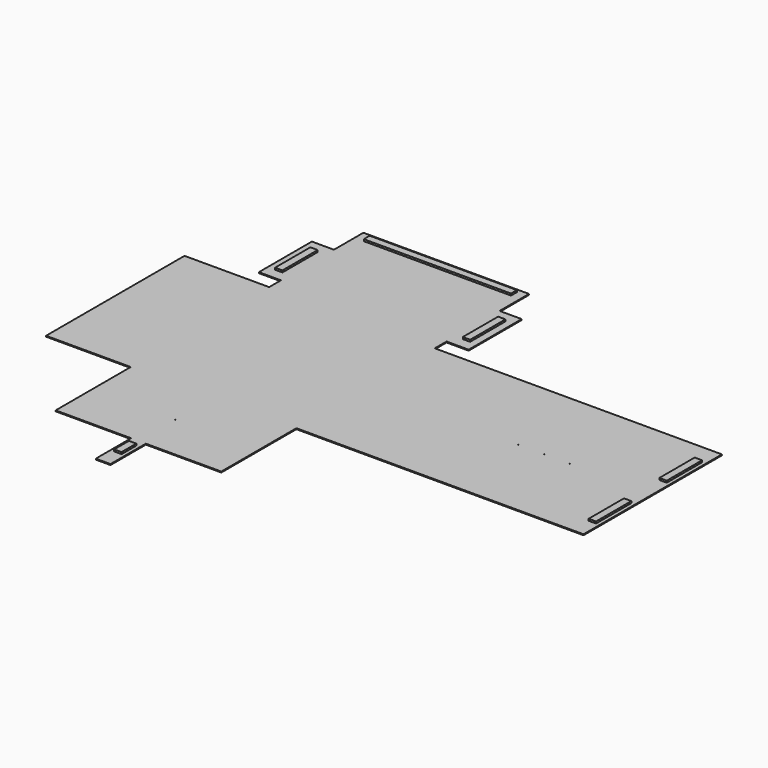
from build123d import *

# Parameters (mm, degrees)
F0_R      = 0.635
F1_DEPTH  = 3.175
F2_W      = 508
F2_H      = 25.4
F3_DEPTH  = 6.35
F4_W      = 25.4
F4_H      = 63.5
F4_H_2    = 152.4
F5_DEPTH  = 6.35
F6_W      = 508
F6_H      = 25.4
F7_DEPTH  = 6.35
F8_W      = 152.4
F8_H      = 25.4
F9_DEPTH  = 6.35
F10_W     = 25.4
F10_H     = 152.4
F11_DEPTH = 6.35
F12_W     = 25.4
F12_H     = 152.4
F13_DEPTH = 6.35
F14_W     = 76.2
F14_H     = 25.4
F15_DEPTH = 6.35


# Not quite as in the source:
# - a feature of the source that left no trace in its solid (it failed there, or was rolled back) is left out


with BuildPart() as f1:
    # F0 (on Top) → F1 (new body)
    with BuildSketch(Plane.XY):
        Polygon((285.75, -298.45), (323.85, -298.45), (577.85, -298.45), (615.95, -298.45), (1187.45, -298.45), (1276.35, -298.45), (1276.35, 298.45), (1187.45, 298.45), (285.75, 298.45), (285.75, 349.25), (361.95, 349.25), (361.95, 577.85), (285.75, 577.85), (285.75, 704.85), (-285.75, 704.85), (-285.75, 577.85), (-361.95, 577.85), (-361.95, 349.25), (-285.75, 349.25), (-285.75, 336.55), (-285.75, 298.45), (-323.85, 298.45), (-361.95, 298.45), (-577.85, 298.45), (-577.85, -298.45), (-323.85, -298.45), (-285.75, -298.45), (-285.75, -336.55), (-285.75, -622.3), (-25.4, -622.3), (-25.4, -774.7), (25.4, -774.7), (25.4, -622.3), (177.8, -622.3), (285.75, -622.3), (285.75, -336.55), align=None)
        with Locations((0, -463.55)):
            Circle(F0_R, mode=Mode.SUBTRACT)
        with Locations((-450.85, 0)):
            Circle(F0_R, mode=Mode.SUBTRACT)
        Circle(F0_R, mode=Mode.SUBTRACT)
        with Locations((0, 463.55)):
            Circle(F0_R, mode=Mode.SUBTRACT)
        with Locations((450.85, 0)):
            Circle(F0_R, mode=Mode.SUBTRACT)
        with Locations((812.8, 0)):
            Circle(F0_R, mode=Mode.SUBTRACT)
        with Locations((901.7, 0)):
            Circle(F0_R, mode=Mode.SUBTRACT)
        with Locations((990.6, 0)):
            Circle(F0_R, mode=Mode.SUBTRACT)
    extrude(amount=F1_DEPTH)

    # F2 (on face) → F3 (join)
    with BuildSketch(Plane.XY.offset(3.175)):
        with Locations((0, 679.45)):
            Rectangle(F2_W, F2_H)
    extrude(amount=F3_DEPTH)

    # F4 (on face) → F5 (join)
    with BuildSketch(Plane.XY.offset(3.175)):
        with Locations((0, -679.45)):
            Rectangle(F4_W, F4_H)
        with Locations((-323.85, 463.55)):
            Rectangle(F4_W, F4_H_2)
        with Locations((323.85, 463.55)):
            Rectangle(F4_W, F4_H_2)
    extrude(amount=F5_DEPTH)

    # F6 (on face) → F7 (join)
    with BuildSketch(Plane(origin=(0, 0, 0), x_dir=(1, 0, 0), z_dir=(0, 0, -1))):
        with Locations((901.7, -247.65)):
            Rectangle(F6_W, F6_H)
    extrude(amount=F7_DEPTH)

    # F8 (on face) → F9 (join)
    with BuildSketch(Plane(origin=(0, 0, 0), x_dir=(1, 0, 0), z_dir=(0, 0, -1))):
        with Locations((450.85, -260.35)):
            Rectangle(F8_W, F8_H)
        with Locations((-450.85, -260.35)):
            Rectangle(F8_W, F8_H)
    extrude(amount=F9_DEPTH)

    # F10 (on face) → F11 (join)
    with BuildSketch(Plane.XY.offset(3.175)):
        with Locations((1250.95, 152.4)):
            Rectangle(F10_W, F10_H)
        with Locations((1250.95, -152.4)):
            Rectangle(F10_W, F10_H)
    extrude(amount=F11_DEPTH)

    # F12 (on face) → F13 (join)
    with BuildSketch(Plane.XY):
        with Locations((-552.45, 152.4)):
            Rectangle(F12_W, F12_H)
        with Locations((-552.45, -152.4)):
            Rectangle(F12_W, F12_H)
    extrude(amount=-F13_DEPTH)

    # F14 (on face) → F15 (join)
    with BuildSketch(Plane(origin=(0, 0, 0), x_dir=(1, 0, 0), z_dir=(0, 0, -1))):
        with Locations((901.7, 247.65)):
            Rectangle(F14_W, F14_H)
    extrude(amount=F15_DEPTH)


solid = f1.part
